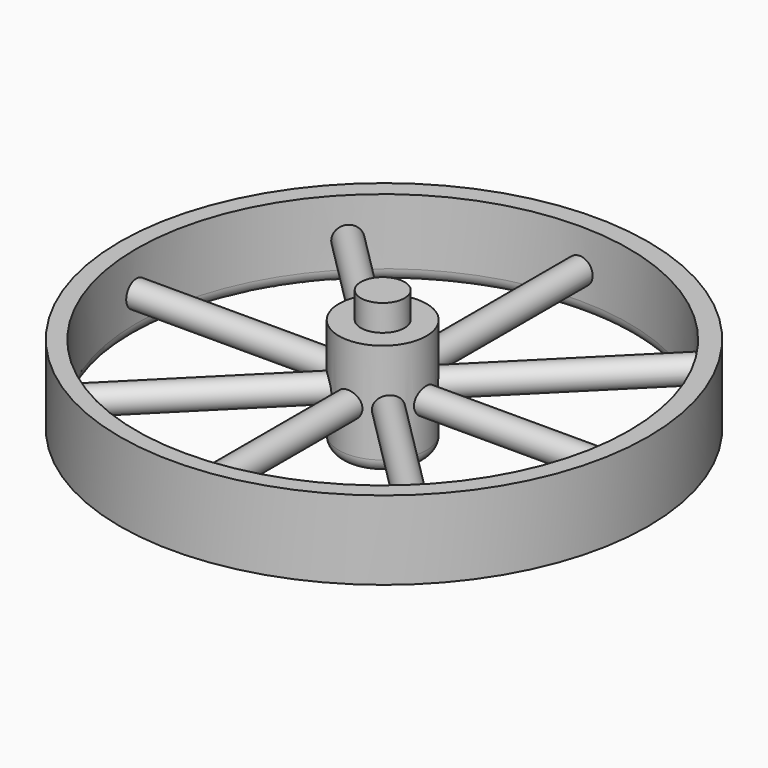
from build123d import *

# Parameters (mm, degrees)
F0_R            = 5
F1_DEPTH        = 6.5
F2_R            = 2.9
F3_DEPTH        = 10
F4_W            = 1.5
F4_H            = 25.2303039929
F5_COPIES_COUNT = 8
F6_R            = 30.1842300119
F6_R_2          = 28.1532988992
F7_DEPTH        = 4.5
F8_R            = 1.5
F9_R            = 2.5
F10_DEPTH       = 3


# Not quite as in the source:
# - a pattern or mirror of a feature is missing from the dataset's text; its kind, count and spacing are read off the source's solid


with BuildPart() as f1:
    # F0 (on Top) → F1 (new body, symmetric)
    with BuildSketch(Plane.XY):
        Circle(F0_R)
    extrude(amount=F1_DEPTH, both=True)

    # F2 (on face) → F3 (cut)
    with BuildSketch(Plane(origin=(0, 0, -6.5), x_dir=(1, 0, 0), z_dir=(0, 0, -1))):
        Circle(F2_R)
    extrude(amount=-F3_DEPTH, mode=Mode.SUBTRACT)

    # F4 (on Top) → F5 (revolve)
    with BuildSketch(Plane.XY):
        with Locations((-0.75, -17.3848480035)):
            Rectangle(F4_W, F4_H)
    f5 = revolve(axis=Axis((0, -23.260904476, 0), (0, -1, 0)))

    # F5_copies: F5 ×8 about axis
    f5_copies_axis = Axis((0, 0, 0), (0, 0, 1))
    for i in range(1, F5_COPIES_COUNT):
        add(f5.rotate(f5_copies_axis, i * 360 / F5_COPIES_COUNT))

    # F6 (on Top) → F7 (join, symmetric)
    with BuildSketch(Plane.XY):
        with Locations((0.0313063833, 0.1453618683)):
            Circle(F6_R)
        Circle(F6_R_2, mode=Mode.SUBTRACT)
    extrude(amount=F7_DEPTH, both=True)

    # F8
    f8_edges = [f1.edges().sort_by_distance(p)[0] for p in [
        (-5, 0, -6.5),
        (-28.153299, 0, -4.5),
    ]]
    fillet(f8_edges, radius=F8_R)

    # F9 (on face) → F10 (join)
    with BuildSketch(Plane.XY.offset(6.5)):
        Circle(F9_R)
    extrude(amount=F10_DEPTH)


solid = f1.part
